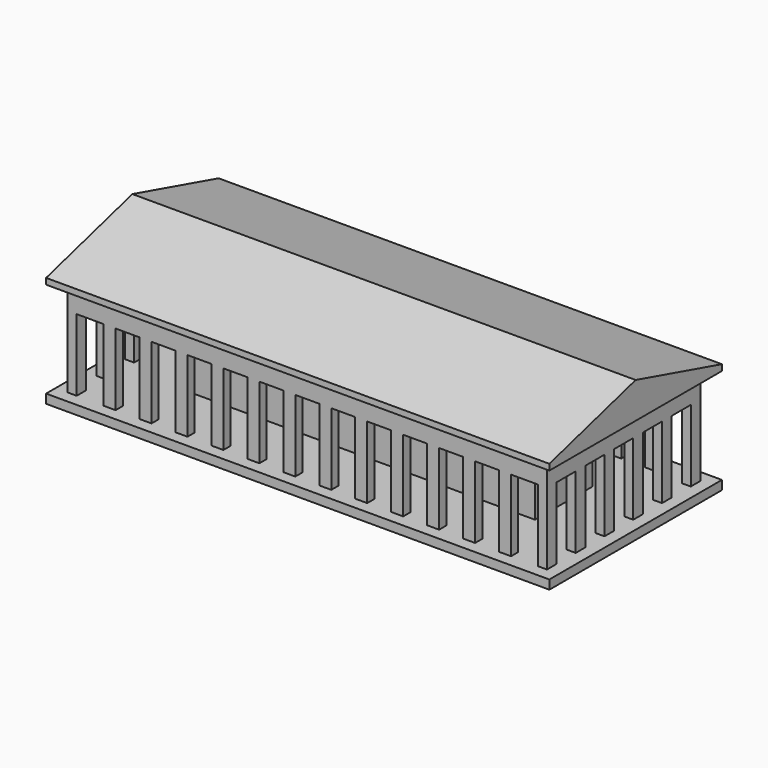
from build123d import *

# Parameters (mm, degrees)
F0_W     = 266.7
F0_H     = 114.3
F1_DEPTH = 4.7752
F2_W     = 4.7625
F2_H     = 6.35
F2_W_2   = 6.35
F2_H_2   = 4.7625
F3_DEPTH = 38.1
F4_W     = 190.5
F4_H     = 38.1
F4_W_2   = 180.975
F4_H_2   = 28.575
F5_DEPTH = 50.8
F6_W     = 254
F6_H     = 101.6
F6_W_2   = 244.475
F6_H_2   = 92.075
F7_DEPTH = 12.7
F9_DEPTH = 266.7


# Not quite as in the source:
# - a feature names something its author has since deleted; it is built from what else it names


with BuildPart() as f1:
    # F0 (on Top) → F1 (new body)
    with BuildSketch(Plane.XY):
        with Locations((-133.35, -57.15)):
            Rectangle(F0_W, F0_H)
    extrude(amount=F1_DEPTH)

    # F2 (on face) → F3 (join)
    with BuildSketch(Plane.XY.offset(4.7752)):
        with Locations((-257.96875, -104.775)):
            Rectangle(F2_W, F2_H)
        with Locations((-257.96875, -85.725)):
            Rectangle(F2_W, F2_H)
        with Locations((-257.96875, -66.675)):
            Rectangle(F2_W, F2_H)
        with Locations((-257.96875, -47.625)):
            Rectangle(F2_W, F2_H)
        with Locations((-257.96875, -28.575)):
            Rectangle(F2_W, F2_H)
        with Locations((-257.96875, -9.525)):
            Rectangle(F2_W, F2_H)
        with Locations((-238.125, -105.56875)):
            Rectangle(F2_W_2, F2_H_2)
        with Locations((-219.075, -105.56875)):
            Rectangle(F2_W_2, F2_H_2)
        with Locations((-200.025, -105.56875)):
            Rectangle(F2_W_2, F2_H_2)
        with Locations((-180.975, -105.56875)):
            Rectangle(F2_W_2, F2_H_2)
        with Locations((-161.925, -105.56875)):
            Rectangle(F2_W_2, F2_H_2)
        with Locations((-142.875, -105.56875)):
            Rectangle(F2_W_2, F2_H_2)
        with Locations((-123.825, -105.56875)):
            Rectangle(F2_W_2, F2_H_2)
        with Locations((-104.775, -105.56875)):
            Rectangle(F2_W_2, F2_H_2)
        with Locations((-85.725, -105.56875)):
            Rectangle(F2_W_2, F2_H_2)
        with Locations((-66.675, -105.56875)):
            Rectangle(F2_W_2, F2_H_2)
        with Locations((-47.625, -105.56875)):
            Rectangle(F2_W_2, F2_H_2)
        with Locations((-28.575, -105.56875)):
            Rectangle(F2_W_2, F2_H_2)
        with Locations((-8.73125, -104.775)):
            Rectangle(F2_W, F2_H)
        with Locations((-8.73125, -85.725)):
            Rectangle(F2_W, F2_H)
        with Locations((-8.73125, -9.525)):
            Rectangle(F2_W, F2_H)
        with Locations((-8.73125, -28.575)):
            Rectangle(F2_W, F2_H)
        with Locations((-8.73125, -47.625)):
            Rectangle(F2_W, F2_H)
        with Locations((-8.73125, -66.675)):
            Rectangle(F2_W, F2_H)
        with Locations((-123.825, -8.73125)):
            Rectangle(F2_W_2, F2_H_2)
        with Locations((-200.025, -8.73125)):
            Rectangle(F2_W_2, F2_H_2)
        with Locations((-180.975, -8.73125)):
            Rectangle(F2_W_2, F2_H_2)
        with Locations((-28.575, -8.73125)):
            Rectangle(F2_W_2, F2_H_2)
        with Locations((-161.925, -8.73125)):
            Rectangle(F2_W_2, F2_H_2)
        with Locations((-238.125, -8.73125)):
            Rectangle(F2_W_2, F2_H_2)
        with Locations((-85.725, -8.73125)):
            Rectangle(F2_W_2, F2_H_2)
        with Locations((-142.875, -8.73125)):
            Rectangle(F2_W_2, F2_H_2)
        with Locations((-66.675, -8.73125)):
            Rectangle(F2_W_2, F2_H_2)
        with Locations((-219.075, -8.73125)):
            Rectangle(F2_W_2, F2_H_2)
        with Locations((-104.775, -8.73125)):
            Rectangle(F2_W_2, F2_H_2)
        with Locations((-47.625, -8.73125)):
            Rectangle(F2_W_2, F2_H_2)
    extrude(amount=F3_DEPTH)

    # F4 (on face) → F5 (join)
    with BuildSketch(Plane.XY.offset(4.7752)):
        with Locations((-133.35, -57.15)):
            Rectangle(F4_W, F4_H)
        with Locations((-133.35, -57.15)):
            Rectangle(F4_W_2, F4_H_2, mode=Mode.SUBTRACT)
    extrude(amount=F5_DEPTH)

    # F6 (on face) → F7 (join)
    with BuildSketch(Plane.XY.offset(42.8752)):
        with Locations((-133.35, -57.15)):
            Rectangle(F6_W, F6_H)
        with Locations((-133.35, -57.15)):
            Rectangle(F6_W_2, F6_H_2, mode=Mode.SUBTRACT)
    extrude(amount=F7_DEPTH)

    # F8 (on face) → F9 (join, through all)
    with BuildSketch(Plane(origin=(-266.7, 0, 0), x_dir=(0, -1, 0), z_dir=(-1, 0, 0))):
        Polygon((0, 58.7502), (114.3, 58.7502), (57.15, 74.6125), align=None)
        Polygon((6.35, 55.5752), (107.95, 55.5752), (114.3, 55.5752), (114.3, 58.7502), (0, 58.7502), (0, 55.5752), align=None)
    extrude(amount=-F9_DEPTH)


solid = f1.part
